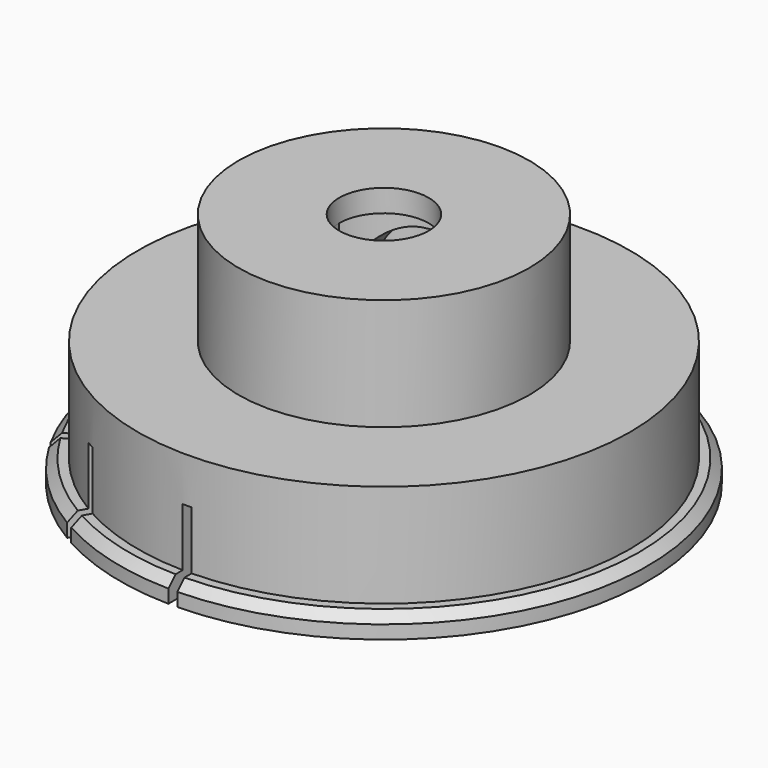
from build123d import *

# Parameters (mm, degrees)
F0_R           = 13.97
F1_DEPTH       = 2.54
F2_R           = 13.97
F2_R_2         = 12.7
F3_DEPTH       = 4.572
F4_R           = 14.986
F4_R_2         = 12.7
F5_DEPTH       = 1.27
F6_SIZE        = 0.508
F8_R           = 6.985
F9_DEPTH       = 7.113
F11_R          = 8.255
F12_DEPTH      = 8.89
F13_R          = 5.842
F14_DEPTH      = 13.463
F15_R          = 2.54
F16_DEPTH      = 1.27
F17_R          = 5.715
F17_R_2        = 4.445
F18_DEPTH      = 7.62
F20_DEPTH      = 14.987
F20_DEPTH_BACK = 14.987
F24_DEPTH      = 1.27
F7_W           = 0.508
F7_H           = 12.703388625
F25_DEPTH      = 4.573


with BuildPart() as f1:
    # F0 (on Top) → F1 (new body)
    with BuildSketch(Plane.XY):
        Circle(F0_R)
    extrude(amount=F1_DEPTH)

    # F2 (on face) → F3 (join)
    with BuildSketch(Plane(origin=(0, 0, 0), x_dir=(1, 0, 0), z_dir=(0, 0, -1))):
        Circle(F2_R)
        Circle(F2_R_2, mode=Mode.SUBTRACT)
    extrude(amount=F3_DEPTH)

    # F4 (on face) → F5 (join)
    with BuildSketch(Plane(origin=(0, 0, -4.572), x_dir=(1, 0, 0), z_dir=(0, 0, -1))):
        Circle(F4_R)
        Circle(F4_R_2, mode=Mode.SUBTRACT)
    extrude(amount=-F5_DEPTH)

    # F6
    f6_edges = [f1.edges().sort_by_distance(p)[0] for p in [
        (-14.986, 0, -3.302),
    ]]
    chamfer(f6_edges, length=F6_SIZE)

    # F8 (on face) → F9 (cut, through all)
    with BuildSketch(Plane.XY.offset(2.54)):
        Circle(F8_R)
    extrude(amount=-F9_DEPTH, mode=Mode.SUBTRACT)

    # F11 (on face) → F12 (join)
    with BuildSketch(Plane(origin=(0, 0, 0), x_dir=(1, 0, 0), z_dir=(0, 0, -1))):
        Circle(F11_R)
        with BuildLine():
            ThreePointArc((-5.4908389692, -2.3146967081), (-6.985, 0), (-5.4908389692, 2.3146967081))
            ThreePointArc((-5.4908389692, 2.3146967081), (-4.913906191, 2.8370450621), (-4.7500056359, 3.5978576814))
            ThreePointArc((-4.7500056359, 3.5978576814), (-3.4925, 6.0491874454), (-0.7408333333, 5.9125543895))
            ThreePointArc((-0.7408333333, 5.9125543895), (0, 5.6740901243), (0.7408333333, 5.9125543895))
            ThreePointArc((0.7408333333, 5.9125543895), (3.4925, 6.0491874454), (4.7500056359, 3.5978576814))
            ThreePointArc((4.7500056359, 3.5978576814), (4.913906191, 2.8370450621), (5.4908389692, 2.3146967081))
            ThreePointArc((5.4908389692, 2.3146967081), (6.985, 0), (5.4908389692, -2.3146967081))
            ThreePointArc((5.4908389692, -2.3146967081), (4.913906191, -2.8370450621), (4.7500056359, -3.5978576814))
            ThreePointArc((4.7500056359, -3.5978576814), (3.4925, -6.0491874454), (0.7408333333, -5.9125543895))
            ThreePointArc((0.7408333333, -5.9125543895), (0, -5.6740901243), (-0.7408333333, -5.9125543895))
            ThreePointArc((-0.7408333333, -5.9125543895), (-3.4925, -6.0491874454), (-4.7500056359, -3.5978576814))
            ThreePointArc((-4.7500056359, -3.5978576814), (-4.913906191, -2.8370450621), (-5.4908389692, -2.3146967081))
        make_face(mode=Mode.SUBTRACT)
    extrude(amount=-F12_DEPTH)

    # F13 (on face) → F14 (cut, through all)
    with BuildSketch(Plane.XY.offset(8.89)):
        Circle(F13_R)
    extrude(amount=-F14_DEPTH, mode=Mode.SUBTRACT)

    # F15 (on face) → F16 (join)
    with BuildSketch(Plane.XY.offset(8.89)):
        with BuildLine():
            ThreePointArc((0.5781535044, -5.813321127), (0.6613572254, -5.8598822935), (0.7408333333, -5.9125543895))
            ThreePointArc((0.7408333333, -5.9125543895), (3.4925, -6.0491874454), (4.7500056359, -3.5978576814))
            ThreePointArc((4.7500056359, -3.5978576814), (4.7441283166, -3.502693305), (4.7454070241, -3.4073561856))
            ThreePointArc((4.7454070241, -3.4073561856), (5.0593204089, -2.921), (5.3235605285, -2.4059649414))
            ThreePointArc((5.3235605285, -2.4059649414), (5.4054855421, -2.3571889885), (5.4908389692, -2.3146967081))
            ThreePointArc((5.4908389692, -2.3146967081), (6.985, 0), (5.4908389692, 2.3146967081))
            ThreePointArc((5.4908389692, 2.3146967081), (5.4054855421, 2.3571889885), (5.3235605285, 2.4059649414))
            ThreePointArc((5.3235605285, 2.4059649414), (5.0593204089, 2.921), (4.7454070241, 3.4073561856))
            ThreePointArc((4.7454070241, 3.4073561856), (4.7441283166, 3.502693305), (4.7500056359, 3.5978576814))
            ThreePointArc((4.7500056359, 3.5978576814), (3.4925, 6.0491874454), (0.7408333333, 5.9125543895))
            ThreePointArc((0.7408333333, 5.9125543895), (0.6613572254, 5.8598822935), (0.5781535044, 5.813321127))
            ThreePointArc((0.5781535044, 5.813321127), (0, 5.842), (-0.5781535044, 5.813321127))
            ThreePointArc((-0.5781535044, 5.813321127), (-0.6613572254, 5.8598822935), (-0.7408333333, 5.9125543895))
            ThreePointArc((-0.7408333333, 5.9125543895), (-3.4925, 6.0491874454), (-4.7500056359, 3.5978576814))
            ThreePointArc((-4.7500056359, 3.5978576814), (-4.7441283166, 3.502693305), (-4.7454070241, 3.4073561856))
            ThreePointArc((-4.7454070241, 3.4073561856), (-5.0593204089, 2.921), (-5.3235605285, 2.4059649414))
            ThreePointArc((-5.3235605285, 2.4059649414), (-5.4054855421, 2.3571889885), (-5.4908389692, 2.3146967081))
            ThreePointArc((-5.4908389692, 2.3146967081), (-6.985, 0), (-5.4908389692, -2.3146967081))
            ThreePointArc((-5.4908389692, -2.3146967081), (-5.4054855421, -2.3571889885), (-5.3235605285, -2.4059649414))
            ThreePointArc((-5.3235605285, -2.4059649414), (-5.0593204089, -2.921), (-4.7454070241, -3.4073561856))
            ThreePointArc((-4.7454070241, -3.4073561856), (-4.7441283166, -3.502693305), (-4.7500056359, -3.5978576814))
            ThreePointArc((-4.7500056359, -3.5978576814), (-3.4925, -6.0491874454), (-0.7408333333, -5.9125543895))
            ThreePointArc((-0.7408333333, -5.9125543895), (-0.6613572254, -5.8598822935), (-0.5781535044, -5.813321127))
            ThreePointArc((-0.5781535044, -5.813321127), (0, -5.842), (0.5781535044, -5.813321127))
        make_face()
        Circle(F15_R, mode=Mode.SUBTRACT)
    extrude(amount=-F16_DEPTH)

    # F7 (on face) → F25 (cut, through all)
    with BuildSketch(Plane(origin=(0, 0, 0), x_dir=(1, 0, 0), z_dir=(0, 0, -1))):
        with Locations((0, 12.6966122789)):
            Rectangle(F7_W, F7_H)
        Polygon((-5.6218601438, 2.9524885306), (-5.3678601438, 3.3924294357), (-16.3693174072, 9.7441237483), (-16.6233174072, 9.3041828431), align=None)
        Polygon((-9.3041828431, 16.6233174072), (-9.7441237483, 16.3693174072), (-3.3924294357, 5.3678601438), (-2.9524885306, 5.6218601438), align=None)
    extrude(amount=F25_DEPTH, mode=Mode.SUBTRACT)


with BuildPart() as f18:
    # F17 (on face) → F18 (new body)
    with BuildSketch(Plane(origin=(0, 0, 7.62), x_dir=(1, 0, 0), z_dir=(0, 0, -1))):
        Circle(F17_R)
        Circle(F17_R_2, mode=Mode.SUBTRACT)
    extrude(amount=F18_DEPTH)

    # F19 (on Front) → F20 (cut, two sides)
    with BuildSketch(Plane.XZ) as f20_sk:
        with BuildLine():
            Line((-1.27, 1.016), (1.27, 1.016))
            ThreePointArc((1.27, 1.016), (3.81, 3.556), (1.27, 6.096))
            Line((1.27, 6.096), (-1.27, 6.096))
            ThreePointArc((-1.27, 6.096), (-3.81, 3.556), (-1.27, 1.016))
        make_face()
    extrude(amount=-F20_DEPTH, mode=Mode.SUBTRACT)
    extrude(f20_sk.sketch, amount=F20_DEPTH_BACK, mode=Mode.SUBTRACT)

    # F23 (on face) → F24 (join)
    with BuildSketch(Plane.XY.offset(7.62)):
        with BuildLine():
            Line((-2.54, 0), (-4.445, 0))
            ThreePointArc((-4.445, 0), (-4.2935402979, -1.1504506555), (-3.8494829198, -2.2225))
            Line((-3.8494829198, -2.2225), (-2.1997045256, -1.27))
            ThreePointArc((-2.1997045256, -1.27), (-2.4534515988, -0.6574003746), (-2.54, 0))
        make_face()
    extrude(amount=-F24_DEPTH)


with BuildPart() as f22:
    # F21 (on Front) → F22 (revolve)
    with BuildSketch(Plane.XZ):
        with BuildLine():
            Line((0, 2.38125), (0, -2.38125))
            ThreePointArc((0, -2.38125), (2.38125, 0), (0, 2.38125))
        make_face()
    revolve(axis=Axis((0, 0, 0), (0, 0, -1)))


solid = Compound([f1.part, f18.part, f22.part])
